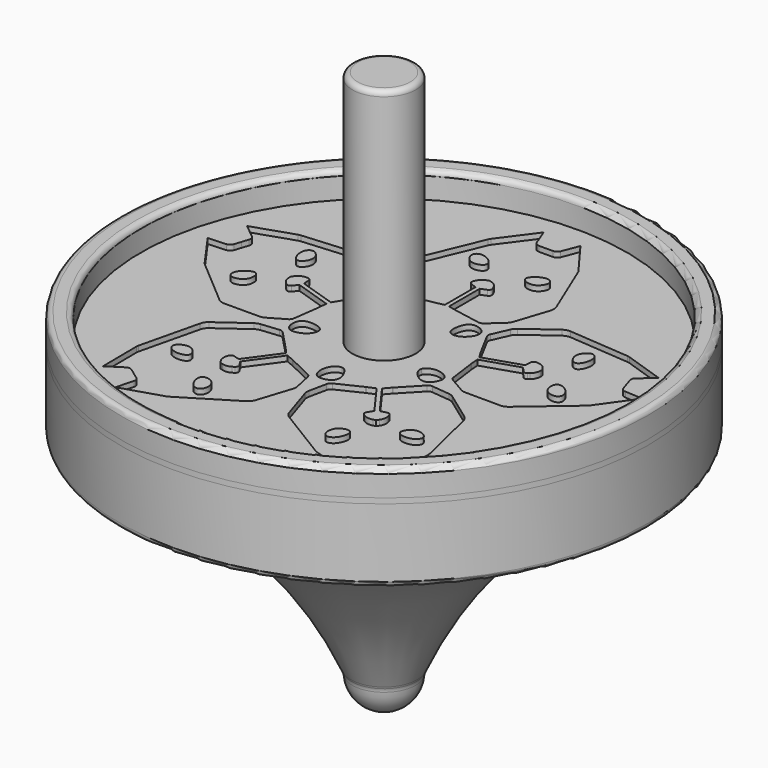
from build123d import *

# Parameters (mm, degrees)
F4_R     = 25
F5_DEPTH = 0.5
F6_DEPTH = 0.5
F7_COUNT = 5


with BuildPart() as f1:
    # F0 (on Front) → F1 (revolve)
    with BuildSketch(Plane.XZ):
        with BuildLine():
            Line((2.5, 20), (0, 20))
            Line((0, 20), (0, -33))
            ThreePointArc((0, -33), (2.0622561718, -32.1787839456), (2.9954737593, -30.1647329878))
            ThreePointArc((2.9954737593, -30.1647329878), (3.0203513187, -29.9914414959), (3.0750690028, -29.8251441441))
            Line((3.0750690028, -29.8251441441), (3.1538549375, -29.6416305562))
            ThreePointArc((3.1538549375, -29.6416305562), (10.3180622492, -18.5626605333), (20.6641236677, -10.3755697008))
            ThreePointArc((20.6641236677, -10.3755697008), (21.3669521344, -10.0954095902), (22.117521619, -10))
            Line((22.117521619, -10), (24.5, -10))
            ThreePointArc((24.5, -10), (24.8535533906, -9.8535533906), (25, -9.5))
            Line((25, -9.5), (25, -3))
            Line((25, -3), (23, -3))
            Line((23, -3), (3, -3))
            Line((3, -3), (3, 19.5))
            ThreePointArc((3, 19.5), (2.8535533906, 19.8535533906), (2.5, 20))
        make_face()
    revolve(axis=Axis((0, 0, -6.5), (0, 0, -1)))

    # F4 (on face) → F6 (cut)
    with BuildSketch(Plane.XY.offset(-3)):
        with BuildLine():
            add(Edge.make_bspline(
                [(2.9697434511, 4.1848174296), (2.7673016741, 4.3175053786), (2.5998920993, 4.9059839494), (3.0594696003, 6.6956649692), (5.2721437306, 5.7727150479), (4.1077092451, 4.0329439669), (3.2020856897, 4.0325315944), (2.9697434511, 4.1848174296)],
                knots=[0, 0, 0, 0, 0.1584389856, 0.3752930049, 0.5942930393, 0.818159724, 1, 1, 1, 1], degree=3))
        make_face()
    extrude(amount=F6_DEPTH, mode=Mode.SUBTRACT)


with BuildPart() as f3:
    # F2 (on Front) → F3 (revolve)
    with BuildSketch(Plane.XZ):
        with BuildLine():
            Line((24.5, 0), (23.5, 0))
            ThreePointArc((23.5, 0), (23.1464466094, -0.1464466094), (23, -0.5))
            Line((23, -0.5), (23, -3))
            Line((23, -3), (25, -3))
            Line((25, -3), (25, -0.5))
            ThreePointArc((25, -0.5), (24.8535533906, -0.1464466094), (24.5, 0))
        make_face()
    revolve(axis=Axis((0, 0, 8.6808623746), (0, 0, -1)))


with BuildPart() as f5:
    # F4 (on face) → F5 (new body)
    with BuildSketch(Plane.XY.offset(-3)):
        Circle(F4_R)
        with BuildLine():
            ThreePointArc((-6.9351535357, -16.7765067987), (-7.0429572028, -16.8337494591), (-7.1569317684, -16.8774318494))
            Line((-7.1569317684, -16.8774318494), (-10.9791679153, -18.0804624426))
            Line((-10.9791679153, -18.0804624426), (-10.5489784736, -16.4464288537))
            ThreePointArc((-10.5489784736, -16.4464288537), (-10.5615478439, -16.1511988144), (-10.7386099607, -15.914623727))
            Line((-10.7386099607, -15.914623727), (-11.2779517934, -15.5227689484))
            Line((-11.2779517934, -15.5227689484), (-11.8172936261, -15.1309141698))
            ThreePointArc((-11.8172936261, -15.1309141698), (-12.0970051077, -15.0356238123), (-12.3816697094, -15.1149007301))
            Line((-12.3816697094, -15.1149007301), (-13.8027921537, -16.0289793503))
            Line((-13.8027921537, -16.0289793503), (-13.8397779947, -12.0220598578))
            ThreePointArc((-13.8397779947, -12.0220598578), (-13.8334536505, -11.9001650036), (-13.8123258104, -11.7799486687))
            Line((-13.8123258104, -11.7799486687), (-12.4707668988, -6.1776344451))
            ThreePointArc((-12.4707668988, -6.1776344451), (-12.3291516716, -5.8540788141), (-12.0838886354, -5.5999348351))
            Line((-12.0838886354, -5.5999348351), (-9.4033690048, -3.6633176085))
            ThreePointArc((-9.4033690048, -3.6633176085), (-9.174087186, -3.5395439083), (-8.9206130671, -3.4792036042))
            Line((-8.9206130671, -3.4792036042), (-7.245987079, -3.3060143064))
            ThreePointArc((-7.245987079, -3.3060143064), (-7.0217216168, -3.334181728), (-6.8327745788, -3.4582277597))
            Line((-6.8327745788, -3.4582277597), (-5.0942783533, -5.2805579852))
            ThreePointArc((-5.0942783533, -5.2805579852), (-5.0785743691, -5.2974034364), (-5.0632624758, -5.3146060603))
            Line((-5.0632624758, -5.3146060603), (-4.543078973, -5.9127514384))
            Line((-4.543078973, -5.9127514384), (-6.6742409995, -8.8460443213))
            Line((-6.6742409995, -8.8460443213), (-7.2611986014, -8.6965142121))
            ThreePointArc((-7.2611986014, -8.6965142121), (-7.4884568034, -8.7292936112), (-7.6259740837, -8.9131679623))
            Line((-7.6259740837, -8.9131679623), (-7.675281362, -9.1067161511))
            ThreePointArc((-7.675281362, -9.1067161511), (-7.6884603978, -9.5412786293), (-7.5159804771, -9.9403637222))
            Line((-7.5159804771, -9.9403637222), (-7.3692310823, -10.1428764295))
            Line((-7.3692310823, -10.1428764295), (-7.1312819955, -10.2198635296))
            ThreePointArc((-7.1312819955, -10.2198635296), (-6.6984302907, -10.2605776061), (-6.28920936, -10.1137564074))
            Line((-6.28920936, -10.1137564074), (-6.1203708808, -10.0070527195))
            ThreePointArc((-6.1203708808, -10.0070527195), (-5.9879911577, -9.8194457146), (-6.0270427431, -9.5931809293))
            Line((-6.0270427431, -9.5931809293), (-6.3506342018, -9.0811584222))
            Line((-6.3506342018, -9.0811584222), (-4.2194721753, -6.1478655393))
            Line((-4.2194721753, -6.1478655393), (-3.4898565732, -6.4577523624))
            ThreePointArc((-3.4898565732, -6.4577523624), (-3.4687642704, -6.4669989352), (-3.4478904962, -6.476728781))
            Line((-3.4478904962, -6.476728781), (-1.1775265822, -7.5670059357))
            ThreePointArc((-1.1775265822, -7.5670059357), (-1.0011639496, -7.7083729156), (-0.9050733006, -7.9129578328))
            Line((-0.9050733006, -7.9129578328), (-0.5522982214, -9.5591402274))
            ThreePointArc((-0.5522982214, -9.5591402274), (-0.5313574503, -9.8188546193), (-0.5782212559, -10.0751627639))
            Line((-0.5782212559, -10.0751627639), (-1.5917275693, -13.2229360603))
            ThreePointArc((-1.5917275693, -13.2229360603), (-1.7576424103, -13.5347298776), (-2.0216005897, -13.7693981509))
            Line((-2.0216005897, -13.7693981509), (-6.9351535357, -16.7765067987))
        make_face(mode=Mode.SUBTRACT)
        with BuildLine():
            add(Edge.make_bspline(
                [(-4.8976990813, -1.5312141568), (-4.9613348703, -1.2976777544), (-5.4692788461, -0.9566119082), (-7.3133839001, -0.8406542357), (-7.1193602725, -3.2302395963), (-5.1049096043, -2.6604154214), (-4.8246643456, -1.7992436679), (-4.8976990813, -1.5312141568)],
                knots=[0, 0, 0, 0, 0.1584389856, 0.3752930049, 0.5942930393, 0.818159724, 1, 1, 1, 1], degree=3))
        make_face(mode=Mode.SUBTRACT)
        with BuildLine():
            add(Edge.make_bspline(
                [(0.0572010478, -5.1311598226), (0.2989719053, -5.1195143372), (0.7803081216, -5.4972026227), (1.4604502227, -7.2152178596), (-0.872137104, -7.7691129102), (-0.9527016001, -5.6771711216), (-0.2202791398, -5.1445253352), (0.0572010478, -5.1311598226)],
                knots=[0, 0, 0, 0, 0.1584389856, 0.3752930049, 0.5942930393, 0.818159724, 1, 1, 1, 1], degree=3))
        make_face(mode=Mode.SUBTRACT)
        with BuildLine():
            ThreePointArc((13.8123258104, -11.7799486687), (13.8334536505, -11.9001650036), (13.8397779947, -12.0220598578))
            Line((13.8397779947, -12.0220598578), (13.8027921537, -16.0289793503))
            Line((13.8027921537, -16.0289793503), (12.3816697094, -15.1149007301))
            ThreePointArc((12.3816697094, -15.1149007301), (12.0970051077, -15.0356238123), (11.8172936261, -15.1309141698))
            Line((11.8172936261, -15.1309141698), (11.2779517934, -15.5227689484))
            Line((11.2779517934, -15.5227689484), (10.7386099607, -15.914623727))
            ThreePointArc((10.7386099607, -15.914623727), (10.5615478439, -16.1511988144), (10.5489784736, -16.4464288537))
            Line((10.5489784736, -16.4464288537), (10.9791679153, -18.0804624426))
            Line((10.9791679153, -18.0804624426), (7.1569317684, -16.8774318494))
            ThreePointArc((7.1569317684, -16.8774318494), (7.0429572028, -16.8337494591), (6.9351535357, -16.7765067987))
            Line((6.9351535357, -16.7765067987), (2.0216005897, -13.7693981509))
            ThreePointArc((2.0216005897, -13.7693981509), (1.7576424103, -13.5347298776), (1.5917275693, -13.2229360603))
            Line((1.5917275693, -13.2229360603), (0.5782212559, -10.0751627639))
            ThreePointArc((0.5782212559, -10.0751627639), (0.5313574503, -9.8188546193), (0.5522982214, -9.5591402274))
            Line((0.5522982214, -9.5591402274), (0.9050733006, -7.9129578328))
            ThreePointArc((0.9050733006, -7.9129578328), (1.0011639496, -7.7083729156), (1.1775265822, -7.5670059357))
            Line((1.1775265822, -7.5670059357), (3.4478904962, -6.476728781))
            ThreePointArc((3.4478904962, -6.476728781), (3.4687642704, -6.4669989352), (3.4898565732, -6.4577523624))
            Line((3.4898565732, -6.4577523624), (4.2194721753, -6.1478655393))
            Line((4.2194721753, -6.1478655393), (6.3506342018, -9.0811584222))
            Line((6.3506342018, -9.0811584222), (6.0270427431, -9.5931809293))
            ThreePointArc((6.0270427431, -9.5931809293), (5.9879911577, -9.8194457146), (6.1203708808, -10.0070527195))
            Line((6.1203708808, -10.0070527195), (6.28920936, -10.1137564074))
            ThreePointArc((6.28920936, -10.1137564074), (6.6984302907, -10.2605776061), (7.1312819955, -10.2198635296))
            Line((7.1312819955, -10.2198635296), (7.3692310823, -10.1428764295))
            Line((7.3692310823, -10.1428764295), (7.5159804771, -9.9403637222))
            ThreePointArc((7.5159804771, -9.9403637222), (7.6884603978, -9.5412786293), (7.675281362, -9.1067161511))
            Line((7.675281362, -9.1067161511), (7.6259740837, -8.9131679623))
            ThreePointArc((7.6259740837, -8.9131679623), (7.4884568034, -8.7292936112), (7.2611986014, -8.6965142121))
            Line((7.2611986014, -8.6965142121), (6.6742409995, -8.8460443213))
            Line((6.6742409995, -8.8460443213), (4.543078973, -5.9127514384))
            Line((4.543078973, -5.9127514384), (5.0632624758, -5.3146060603))
            ThreePointArc((5.0632624758, -5.3146060603), (5.0785743691, -5.2974034364), (5.0942783533, -5.2805579852))
            Line((5.0942783533, -5.2805579852), (6.8327745788, -3.4582277597))
            ThreePointArc((6.8327745788, -3.4582277597), (7.0217216168, -3.334181728), (7.245987079, -3.3060143064))
            Line((7.245987079, -3.3060143064), (8.9206130671, -3.4792036042))
            ThreePointArc((8.9206130671, -3.4792036042), (9.174087186, -3.5395439083), (9.4033690048, -3.6633176085))
            Line((9.4033690048, -3.6633176085), (12.0838886354, -5.5999348351))
            ThreePointArc((12.0838886354, -5.5999348351), (12.3291516716, -5.8540788141), (12.4707668988, -6.1776344451))
            Line((12.4707668988, -6.1776344451), (13.8123258104, -11.7799486687))
        make_face(mode=Mode.SUBTRACT)
        with BuildLine():
            add(Edge.make_bspline(
                [(4.8623468896, -1.6400170153), (4.7765600711, -1.8663561119), (4.9870219053, -2.4408461557), (6.0648897479, -3.3324736334), (6.6648216484, -2.9189230724), (6.792586925, -2.778554323)],
                knots=[0, 0, 0, 0, 0.1584389856, 0.3752930049, 0.4499157178, 0.4499157178, 0.4499157178, 0.4499157178], degree=3))
            add(Edge.make_bspline(
                [(6.792586925, -2.778554323), (7.0397825532, -2.5069739524), (7.4236875204, -1.4849642044), (5.6937115743, -0.8482692917), (4.960804341, -1.3802478452), (4.8623468896, -1.6400170153)],
                knots=[0.4499157178, 0.4499157178, 0.4499157178, 0.4499157178, 0.5942930393, 0.818159724, 1, 1, 1, 1], degree=3))
        make_face(mode=Mode.SUBTRACT)
        with BuildLine():
            ThreePointArc((-18.0984864127, 1.4114972546), (-18.1862405831, 1.4963356798), (-18.2630050827, 1.5912333321))
            Line((-18.2630050827, 1.5912333321), (-20.5882910936, 4.8546390285))
            Line((-20.5882910936, 4.8546390285), (-18.9012969527, 4.950448705))
            ThreePointArc((-18.9012969527, 4.950448705), (-18.6244006491, 5.0536339859), (-18.4541195737, 5.2951357883))
            Line((-18.4541195737, 5.2951357883), (-18.2481093252, 5.9291701388))
            Line((-18.2481093252, 5.9291701388), (-18.0420990766, 6.5632044892))
            ThreePointArc((-18.0420990766, 6.5632044892), (-18.0379081626, 6.8586722563), (-18.2012711915, 7.1049064659))
            Line((-18.2012711915, 7.1049064659), (-19.509762606, 8.1740083992))
            Line((-19.509762606, 8.1740083992), (-15.7103849658, 9.4473902424))
            ThreePointArc((-15.7103849658, 9.4473902424), (-15.5925017406, 9.4790430152), (-15.4716403503, 9.4960981357))
            Line((-15.4716403503, 9.4960981357), (-9.7289583989, 9.9514100938))
            ThreePointArc((-9.7289583989, 9.9514100938), (-9.3774771958, 9.9167101977), (-9.0599814622, 9.7619859974))
            Line((-9.0599814622, 9.7619859974), (-6.3898229097, 7.8111079703))
            ThreePointArc((-6.3898229097, 7.8111079703), (-6.201255147, 7.6312961793), (-6.0655402973, 7.4088741462))
            Line((-6.0655402973, 7.4088741462), (-5.3833395975, 5.8697286242))
            ThreePointArc((-5.3833395975, 5.8697286242), (-5.3408265683, 5.647735283), (-5.4004135093, 5.4297036393))
            Line((-5.4004135093, 5.4297036393), (-6.5963276668, 3.2131644666))
            ThreePointArc((-6.5963276668, 3.2131644666), (-6.6074958449, 3.1930235593), (-6.6191248772, 3.1731451803))
            Line((-6.6191248772, 3.1731451803), (-7.0272493942, 2.4935841834))
            Line((-7.0272493942, 2.4935841834), (-10.4755419886, 3.6140023657))
            Line((-10.4755419886, 3.6140023657), (-10.5147102778, 4.2184395626))
            ThreePointArc((-10.5147102778, 4.2184395626), (-10.6161119855, 4.4244455651), (-10.8334820619, 4.4984119714))
            Line((-10.8334820619, 4.4984119714), (-11.032794115, 4.4854963001))
            ThreePointArc((-11.032794115, 4.4854963001), (-11.4501601376, 4.3637431171), (-11.7764133892, 4.0763808887))
            Line((-11.7764133892, 4.0763808887), (-11.9236663621, 3.8742340524))
            Line((-11.9236663621, 3.8742340524), (-11.9233551338, 3.6241407006))
            ThreePointArc((-11.9233551338, 3.6241407006), (-11.8283179887, 3.1998929245), (-11.5622265089, 2.8560709374))
            Line((-11.5622265089, 2.8560709374), (-11.4085713118, 2.7284692544))
            ThreePointArc((-11.4085713118, 2.7284692544), (-11.1892388632, 2.6605424088), (-10.9861158683, 2.7676023375))
            Line((-10.9861158683, 2.7676023375), (-10.5991487864, 3.2335797591))
            Line((-10.5991487864, 3.2335797591), (-7.1508561919, 2.1131615768))
            Line((-7.1508561919, 2.1131615768), (-7.2201124539, 1.3234956095))
            ThreePointArc((-7.2201124539, 1.3234956095), (-7.2223885872, 1.3005782893), (-7.2251918695, 1.2777194626))
            Line((-7.2251918695, 1.2777194626), (-7.5605260292, -1.2184391016))
            ThreePointArc((-7.5605260292, -1.2184391016), (-7.640474966, -1.4298547318), (-7.8053531411, -1.5844625859))
            Line((-7.8053531411, -1.5844625859), (-9.2619521398, -2.4286699595))
            ThreePointArc((-9.2619521398, -2.4286699595), (-9.5024841505, -2.5288419771), (-9.760729394, -2.5634754218))
            Line((-9.760729394, -2.5634754218), (-13.067630374, -2.5722890813))
            ThreePointArc((-13.067630374, -2.5722890813), (-13.4154344212, -2.5108442788), (-13.7201847749, -2.3323216168))
            Line((-13.7201847749, -2.3323216168), (-18.0984864127, 1.4114972546))
        make_face(mode=Mode.SUBTRACT)
        with BuildLine():
            add(Edge.make_bspline(
                [(-2.9697434511, 4.1848174296), (-2.7673016741, 4.3175053786), (-2.5998920993, 4.9059839494), (-3.0594696003, 6.6956649692), (-5.2721437306, 5.7727150479), (-4.1077092451, 4.0329439669), (-3.2020856897, 4.0325315944), (-2.9697434511, 4.1848174296)],
                knots=[0, 0, 0, 0, 0.1584389856, 0.3752930049, 0.5942930393, 0.818159724, 1, 1, 1, 1], degree=3))
        make_face(mode=Mode.SUBTRACT)
        with BuildLine():
            ThreePointArc((-2.8531695489, 0.9270509831), (-1.7633557569, 2.4270509831), (0, 3))
            ThreePointArc((0, 3), (1.7633557569, 2.4270509831), (2.8531695489, 0.9270509831))
            ThreePointArc((2.8531695489, 0.9270509831), (2.9630650218, 0.4693033951), (3, 0))
            ThreePointArc((3, 0), (2.6730195726, -1.3619714992), (1.7633557569, -2.4270509831))
            ThreePointArc((1.7633557569, -2.4270509831), (0, -3), (-1.7633557569, -2.4270509831))
            ThreePointArc((-1.7633557569, -2.4270509831), (-2.8531695489, -0.9270509831), (-2.8531695489, 0.9270509831))
        make_face(mode=Mode.SUBTRACT)
        with BuildLine():
            add(Edge.make_bspline(
                [(2.9697434511, 4.1848174296), (2.7673016741, 4.3175053786), (2.5998920993, 4.9059839494), (3.0594696003, 6.6956649692), (5.2721437306, 5.7727150479), (4.1077092451, 4.0329439669), (3.2020856897, 4.0325315944), (2.9697434511, 4.1848174296)],
                knots=[0, 0, 0, 0, 0.1584389856, 0.3752930049, 0.5942930393, 0.818159724, 1, 1, 1, 1], degree=3))
        make_face(mode=Mode.SUBTRACT)
        with BuildLine():
            ThreePointArc((15.4716403503, 9.4960981357), (15.5925017406, 9.4790430152), (15.7103849658, 9.4473902424))
            Line((15.7103849658, 9.4473902424), (19.509762606, 8.1740083992))
            Line((19.509762606, 8.1740083992), (18.2012711915, 7.1049064659))
            ThreePointArc((18.2012711915, 7.1049064659), (18.0379081626, 6.8586722563), (18.0420990766, 6.5632044892))
            Line((18.0420990766, 6.5632044892), (18.2481093252, 5.9291701388))
            Line((18.2481093252, 5.9291701388), (18.4541195737, 5.2951357883))
            ThreePointArc((18.4541195737, 5.2951357883), (18.6244006491, 5.0536339859), (18.9012969527, 4.950448705))
            Line((18.9012969527, 4.950448705), (20.5882910936, 4.8546390285))
            Line((20.5882910936, 4.8546390285), (18.2630050827, 1.5912333321))
            ThreePointArc((18.2630050827, 1.5912333321), (18.1862405831, 1.4963356798), (18.0984864127, 1.4114972546))
            Line((18.0984864127, 1.4114972546), (13.7201847749, -2.3323216168))
            ThreePointArc((13.7201847749, -2.3323216168), (13.4154344212, -2.5108442788), (13.067630374, -2.5722890813))
            Line((13.067630374, -2.5722890813), (9.760729394, -2.5634754218))
            ThreePointArc((9.760729394, -2.5634754218), (9.5024841505, -2.5288419771), (9.2619521398, -2.4286699595))
            Line((9.2619521398, -2.4286699595), (7.8053531411, -1.5844625859))
            ThreePointArc((7.8053531411, -1.5844625859), (7.640474966, -1.4298547318), (7.5605260292, -1.2184391016))
            Line((7.5605260292, -1.2184391016), (7.2251918695, 1.2777194626))
            ThreePointArc((7.2251918695, 1.2777194626), (7.2223885872, 1.3005782893), (7.2201124539, 1.3234956095))
            Line((7.2201124539, 1.3234956095), (7.1508561919, 2.1131615768))
            Line((7.1508561919, 2.1131615768), (10.5991487864, 3.2335797591))
            Line((10.5991487864, 3.2335797591), (10.9861158683, 2.7676023375))
            ThreePointArc((10.9861158683, 2.7676023375), (11.1892388632, 2.6605424088), (11.4085713118, 2.7284692544))
            Line((11.4085713118, 2.7284692544), (11.5622265089, 2.8560709374))
            ThreePointArc((11.5622265089, 2.8560709374), (11.8283179887, 3.1998929245), (11.9233551338, 3.6241407006))
            Line((11.9233551338, 3.6241407006), (11.9236663621, 3.8742340524))
            Line((11.9236663621, 3.8742340524), (11.7764133892, 4.0763808887))
            ThreePointArc((11.7764133892, 4.0763808887), (11.4501601376, 4.3637431171), (11.032794115, 4.4854963001))
            Line((11.032794115, 4.4854963001), (10.8334820619, 4.4984119714))
            ThreePointArc((10.8334820619, 4.4984119714), (10.6161119855, 4.4244455651), (10.5147102778, 4.2184395626))
            Line((10.5147102778, 4.2184395626), (10.4755419886, 3.6140023657))
            Line((10.4755419886, 3.6140023657), (7.0272493942, 2.4935841834))
            Line((7.0272493942, 2.4935841834), (6.6191248772, 3.1731451803))
            ThreePointArc((6.6191248772, 3.1731451803), (6.6074958449, 3.1930235593), (6.5963276668, 3.2131644666))
            Line((6.5963276668, 3.2131644666), (5.4004135093, 5.4297036393))
            ThreePointArc((5.4004135093, 5.4297036393), (5.3408265683, 5.647735283), (5.3833395975, 5.8697286242))
            Line((5.3833395975, 5.8697286242), (6.0655402973, 7.4088741462))
            ThreePointArc((6.0655402973, 7.4088741462), (6.201255147, 7.6312961793), (6.3898229097, 7.8111079703))
            Line((6.3898229097, 7.8111079703), (9.0599814622, 9.7619859974))
            ThreePointArc((9.0599814622, 9.7619859974), (9.3774771958, 9.9167101977), (9.7289583989, 9.9514100938))
            Line((9.7289583989, 9.9514100938), (15.4716403503, 9.4960981357))
        make_face(mode=Mode.SUBTRACT)
        with BuildLine():
            Line((0.9724183259, 7.275717633), (0.2, 7.4538712175))
            Line((0.2, 7.4538712175), (0.2, 11.0796206187))
            Line((0.2, 11.0796206187), (0.7627502679, 11.3036532412))
            ThreePointArc((0.7627502679, 11.3036532412), (0.927338768, 11.4637513518), (0.930513953, 11.693339456))
            Line((0.930513953, 11.693339456), (0.8566396081, 11.8789053209))
            ThreePointArc((0.8566396081, 11.8789053209), (0.6118722561, 12.2382201938), (0.2377567371, 12.4597056625))
            Line((0.2377567371, 12.4597056625), (0, 12.5372847542))
            Line((0, 12.5372847542), (-0.2377567371, 12.4597056625))
            ThreePointArc((-0.2377567371, 12.4597056625), (-0.6118722561, 12.2382201938), (-0.8566396081, 11.8789053209))
            Line((-0.8566396081, 11.8789053209), (-0.930513953, 11.693339456))
            ThreePointArc((-0.930513953, 11.693339456), (-0.927338768, 11.4637513518), (-0.7627502679, 11.3036532412))
            Line((-0.7627502679, 11.3036532412), (-0.2, 11.0796206187))
            Line((-0.2, 11.0796206187), (-0.2, 7.4538712175))
            Line((-0.2, 7.4538712175), (-0.9724183259, 7.275717633))
            ThreePointArc((-0.9724183259, 7.275717633), (-0.9949173565, 7.270800523), (-1.0175236544, 7.266402837))
            Line((-1.0175236544, 7.266402837), (-3.4951354767, 6.8139691577))
            ThreePointArc((-3.4951354767, 6.8139691577), (-3.7209092696, 6.8246740924), (-3.9189002348, 6.9337061009))
            Line((-3.9189002348, 6.9337061009), (-5.1719030032, 8.058139645))
            ThreePointArc((-5.1719030032, 8.058139645), (-5.3415007322, 8.2559443253), (-5.4542412645, 8.4908478239))
            Line((-5.4542412645, 8.4908478239), (-6.4845121543, 11.6331739792))
            ThreePointArc((-6.4845121543, 11.6331739792), (-6.5335520359, 11.9829427728), (-6.4579399332, 12.327944119))
            Line((-6.4579399332, 12.327944119), (-4.2503262123, 17.6488600771))
            ThreePointArc((-4.2503262123, 17.6488600771), (-4.1967576051, 17.7585357678), (-4.1302261094, 17.8608681326))
            Line((-4.1302261094, 17.8608681326), (-1.7450957508, 21.0807943653))
            Line((-1.7450957508, 21.0807943653), (-1.1326654747, 19.5059744129))
            ThreePointArc((-1.1326654747, 19.5059744129), (-0.9489647773, 19.2745163844), (-0.6666631683, 19.1871976192))
            Line((-0.6666631683, 19.1871976192), (0, 19.1871976192))
            Line((0, 19.1871976192), (0.6666631683, 19.1871976192))
            ThreePointArc((0.6666631683, 19.1871976192), (0.9489647773, 19.2745163844), (1.1326654747, 19.5059744129))
            Line((1.1326654747, 19.5059744129), (1.7450957508, 21.0807943653))
            Line((1.7450957508, 21.0807943653), (4.1302261094, 17.8608681326))
            ThreePointArc((4.1302261094, 17.8608681326), (4.1967576051, 17.7585357678), (4.2503262123, 17.6488600771))
            Line((4.2503262123, 17.6488600771), (6.4579399332, 12.327944119))
            ThreePointArc((6.4579399332, 12.327944119), (6.5335520359, 11.9829427728), (6.4845121543, 11.6331739792))
            Line((6.4845121543, 11.6331739792), (5.4542412645, 8.4908478239))
            ThreePointArc((5.4542412645, 8.4908478239), (5.3415007322, 8.2559443253), (5.1719030032, 8.058139645))
            Line((5.1719030032, 8.058139645), (3.9189002348, 6.9337061009))
            ThreePointArc((3.9189002348, 6.9337061009), (3.7209092696, 6.8246740924), (3.4951354767, 6.8139691577))
            Line((3.4951354767, 6.8139691577), (1.0175236544, 7.266402837))
            ThreePointArc((1.0175236544, 7.266402837), (0.9949173565, 7.270800523), (0.9724183259, 7.275717633))
        make_face(mode=Mode.SUBTRACT)
    extrude(amount=F5_DEPTH)


with BuildPart() as f5b:
    # F4 (on face) → F5, piece 2 (new body)
    with BuildSketch(Plane.XY.offset(-3)):
        with BuildLine():
            add(Edge.make_bspline(
                [(-1.8467439804, 14.443160966), (-1.7744591949, 14.7946883369), (-2.7551902834, 15.6573196595), (-3.9676321919, 15.2276031184), (-3.1472779832, 13.6710523116), (-1.9147193977, 14.1125904376), (-1.8467439804, 14.443160966)],
                knots=[0, 0, 0, 0, 0.2702066563, 0.4881898307, 0.7459021273, 1, 1, 1, 1], degree=3))
        make_face()
    extrude(amount=F5_DEPTH)


with BuildPart() as f5c:
    # F4 (on face) → F5, piece 3 (new body)
    with BuildSketch(Plane.XY.offset(-3)):
        with BuildLine():
            add(Edge.make_bspline(
                [(1.8467439804, 14.443160966), (1.7744591949, 14.7946883369), (2.7551902834, 15.6573196595), (3.9676321919, 15.2276031184), (3.1472779832, 13.6710523116), (1.9147193977, 14.1125904376), (1.8467439804, 14.443160966)],
                knots=[0, 0, 0, 0, 0.2702066563, 0.4881898307, 0.7459021273, 1, 1, 1, 1], degree=3))
        make_face()
    extrude(amount=F5_DEPTH)


with BuildPart() as f7_1:
    # F7: instance of F5b
    add(f5b.part.rotate(Axis((0, 0, -6.5), (0, 0, -1)), 1 * 360 / F7_COUNT))


with BuildPart() as f7_2:
    # F7: instance of F5b
    add(f5b.part.rotate(Axis((0, 0, -6.5), (0, 0, -1)), 2 * 360 / F7_COUNT))


with BuildPart() as f7_3:
    # F7: instance of F5b
    add(f5b.part.rotate(Axis((0, 0, -6.5), (0, 0, -1)), 3 * 360 / F7_COUNT))


with BuildPart() as f7_4:
    # F7: instance of F5b
    add(f5b.part.rotate(Axis((0, 0, -6.5), (0, 0, -1)), 4 * 360 / F7_COUNT))


with BuildPart() as f7_5:
    # F7: instance of F5c
    add(f5c.part.rotate(Axis((0, 0, -6.5), (0, 0, -1)), 1 * 360 / F7_COUNT))


with BuildPart() as f7_6:
    # F7: instance of F5c
    add(f5c.part.rotate(Axis((0, 0, -6.5), (0, 0, -1)), 2 * 360 / F7_COUNT))


with BuildPart() as f7_7:
    # F7: instance of F5c
    add(f5c.part.rotate(Axis((0, 0, -6.5), (0, 0, -1)), 3 * 360 / F7_COUNT))


with BuildPart() as f7_8:
    # F7: instance of F5c
    add(f5c.part.rotate(Axis((0, 0, -6.5), (0, 0, -1)), 4 * 360 / F7_COUNT))


solid = Compound([f1.part, f3.part, f5.part, f5b.part, f5c.part, f7_1.part, f7_2.part, f7_3.part, f7_4.part, f7_5.part, f7_6.part, f7_7.part, f7_8.part])
